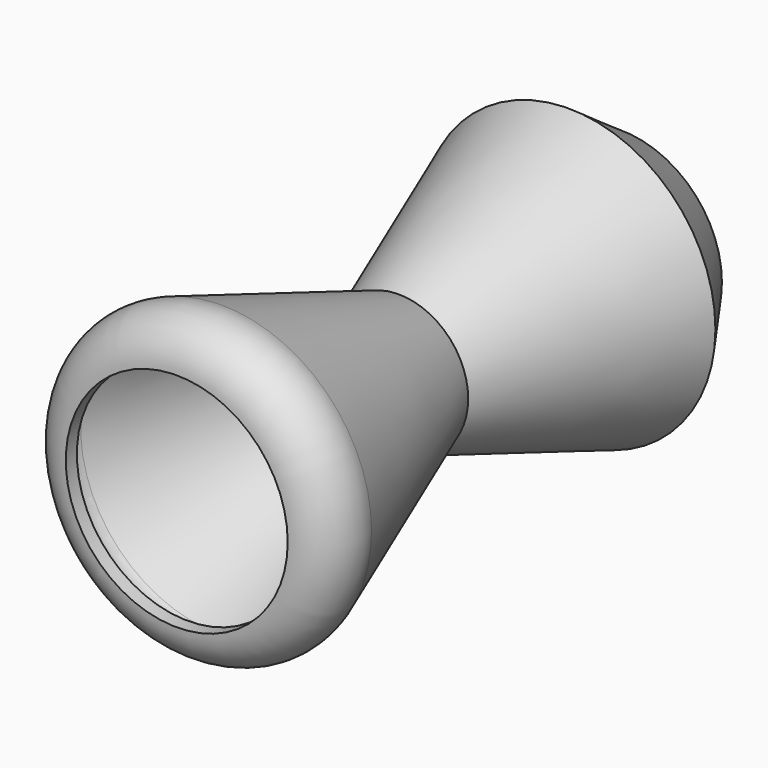
from build123d import *

# Parameters (mm, degrees)
F0_R      = 63.5
F1_DEPTH  = 254
F1_TAPER  = -20
F1_FACE_R = 63.5
F2_DEPTH  = 254
F2_TAPER  = -20
F3_R      = 38.1
F5_T      = -12.7


# Not quite as in the source:
# - a fillet or chamfer that OpenCascade refuses, or shapes differently, is made with other operations: its cross-section is extruded or revolved along the edge and cut away or added
# - a shell that OpenCascade refuses in one call is made with other operations: the cavity is built on its own and cut out


with BuildPart() as f1:
    # F0 (on Front) → F1 (new body)
    with BuildSketch(Plane.XZ):
        Circle(F0_R)
    extrude(amount=F1_DEPTH, taper=F1_TAPER)

    # F1_face (on face) → F2 (join)
    with BuildSketch(Plane(origin=(0, 0, 0), x_dir=(1, 0, 0), z_dir=(0, 1, 0))):
        Circle(F1_FACE_R)
    extrude(amount=F2_DEPTH, taper=F2_TAPER)

    # F3
    f3_edges = [f1.edges().sort_by_distance(p)[0] for p in [
        (-155.94844, -254, 0),
    ]]
    fillet(f3_edges, radius=F3_R)

    # F4: chamfer of 63.5 on 1 edges, made by hand

    # F4_s1 → F4_t2 (revolve, cut)
    with BuildSketch(Plane.XY):
        Polygon((134.2301604024, 194.3295185801), (92.4484395036, 254), (155.9484395036, 254), align=None)
    revolve(axis=Axis((0, 254, 0), (0, -1, 0)), mode=Mode.SUBTRACT)

    # F5: a shell. OpenCascade refuses it in one call, so the cavity is built on its own and cut out:
    # the body offset inwards by the wall thickness, plus a prism from it out through each open face.
    f5_core = offset(f1.part, amount=F5_T, kind=Kind.INTERSECTION, mode=Mode.PRIVATE)
    f5_exits = [f5_core.faces().sort_by_distance(p)[0] for p in [
        (0, -241.3, 0),
    ]]
    add(f5_core, mode=Mode.SUBTRACT)
    extrude(f5_exits, amount=-F5_T, mode=Mode.SUBTRACT)


solid = f1.part
